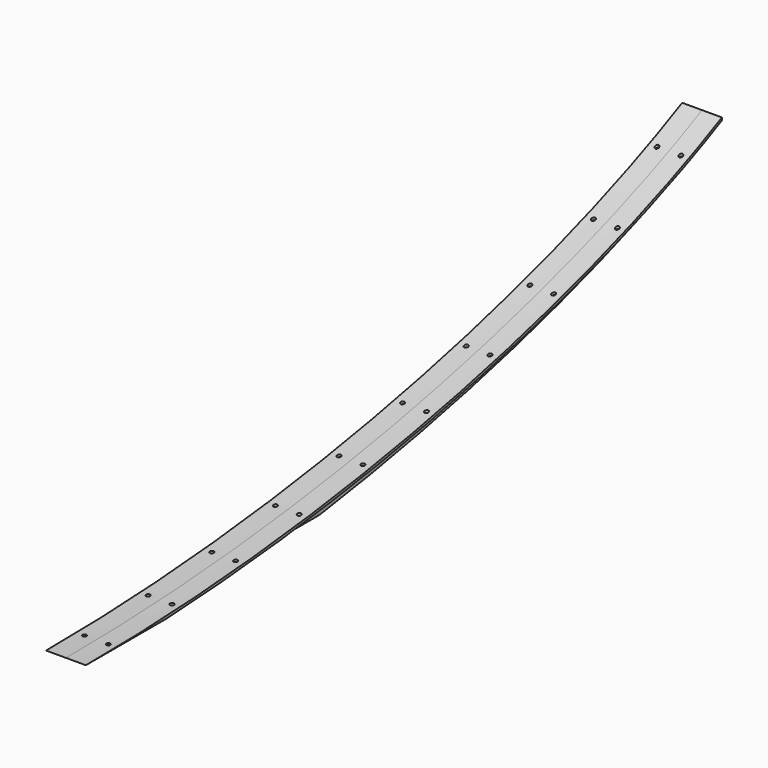
from build123d import *

# Parameters (mm, degrees)
F1_DEPTH = 25
F2_DEPTH = 4.5
F3_DEPTH = 1.5
F4_R     = 2.5
F5_DEPTH = 150
F6_R     = 4.1800646045
F7_DEPTH = 12.5


# Not quite as in the source:
# - the dataset's text gives a spline's control points without its knots; the knots are read off the source's solid


with BuildPart() as f1:
    # F0 (on Right) → F1 (new body, symmetric)
    with BuildSketch(Plane.YZ):
        with BuildLine():
            add(Edge.make_bspline(
                [(-542.9529296271, -39.9508323044), (-188.0693441655, -39.9508323044), (204.5968802247, 34.2876766354), (457.0470703729, 160.0491676956)],
                knots=[0, 0, 0, 0, 1019.8039027186, 1019.8039027186, 1019.8039027186, 1019.8039027186], degree=3))
            Line((-542.9529296271, -39.9508323044), (-417.3127151335, -39.9508323044))
            add(Edge.make_bspline(
                [(-417.3127151335, -39.9508323044), (-369.1001563129, -37.6799090107), (-229.605831227, -27.4883990926), (-0.7659143619, 6.0089411279), (250.4802761754, 69.14721948), (394.0857076642, 125.4398419701), (457.047070373, 156.6986558412)],
                knots=[0.116693999, 0.116693999, 0.116693999, 0.116693999, 0.25, 0.5, 0.75, 0.9982402372, 0.9982402372, 0.9982402372, 0.9982402372], degree=3))
            Line((457.0470703729, 156.6986558412), (457.0470703729, 160.0491676956))
        make_face()
    extrude(amount=F1_DEPTH, both=True)

    # F0 (on Right) → F2 (join, symmetric)
    with BuildSketch(Plane.YZ):
        with BuildLine():
            add(Edge.make_bspline(
                [(-417.3127151335, -39.9508323044), (-369.1001563129, -37.6799090107), (-229.605831227, -27.4883990926), (-0.7659143619, 6.0089411279), (250.4802761754, 69.14721948), (394.0857076642, 125.4398419701), (457.047070373, 156.6986558412)],
                knots=[0.116693999, 0.116693999, 0.116693999, 0.116693999, 0.25, 0.5, 0.75, 0.9982402372, 0.9982402372, 0.9982402372, 0.9982402372], degree=3))
            Line((-417.3127151335, -39.9508323044), (-149.937543661, -39.9508323044))
            add(Edge.make_bspline(
                [(-149.937543661, -39.9508323044), (-98.996798705, -32.7943859429), (-3.7016307054, -16.778446645), (131.246444394, 13.3933570474), (254.1058325956, 48.1234806847), (363.3774188375, 86.6936370443), (428.3490574687, 114.995507991), (457.0470703729, 128.861665731)],
                knots=[0.3594995159, 0.3594995159, 0.3594995159, 0.3594995159, 0.5, 0.625, 0.75, 0.875, 0.9840561675, 0.9840561675, 0.9840561675, 0.9840561675], degree=3))
            Line((457.0470703729, 128.861665731), (457.0470703729, 156.6986558412))
        make_face()
    extrude(amount=F2_DEPTH, both=True)

    # F0 (on Right) → F3 (cut, symmetric)
    with BuildSketch(Plane.YZ):
        with BuildLine():
            add(Edge.make_bspline(
                [(-417.3127151335, -39.9508323044), (-369.1001563129, -37.6799090107), (-229.605831227, -27.4883990926), (-0.7659143619, 6.0089411279), (250.4802761754, 69.14721948), (394.0857076642, 125.4398419701), (457.047070373, 156.6986558412)],
                knots=[0.116693999, 0.116693999, 0.116693999, 0.116693999, 0.25, 0.5, 0.75, 0.9982402372, 0.9982402372, 0.9982402372, 0.9982402372], degree=3))
            Line((-417.3127151335, -39.9508323044), (-149.937543661, -39.9508323044))
            add(Edge.make_bspline(
                [(-149.937543661, -39.9508323044), (-98.996798705, -32.7943859429), (-3.7016307054, -16.778446645), (131.246444394, 13.3933570474), (254.1058325956, 48.1234806847), (363.3774188375, 86.6936370443), (428.3490574687, 114.995507991), (457.0470703729, 128.861665731)],
                knots=[0.3594995159, 0.3594995159, 0.3594995159, 0.3594995159, 0.5, 0.625, 0.75, 0.875, 0.9840561675, 0.9840561675, 0.9840561675, 0.9840561675], degree=3))
            Line((457.0470703729, 128.861665731), (457.0470703729, 156.6986558412))
        make_face()
    extrude(amount=F3_DEPTH, both=True, mode=Mode.SUBTRACT)

    # F4 (on Top) → F5 (cut, symmetric)
    with BuildSketch(Plane.XY):
        with Locations((15, -494.9529296271)):
            Circle(F4_R)
        with Locations((15, -394.9529296271)):
            Circle(F4_R)
        with Locations((15, -294.9529296271)):
            Circle(F4_R)
        with Locations((15, -194.9529296271)):
            Circle(F4_R)
        with Locations((15, -94.9529296271)):
            Circle(F4_R)
        with Locations((15, 5.0470703729)):
            Circle(F4_R)
        with Locations((15, 105.0470703729)):
            Circle(F4_R)
        with Locations((15, 205.0470703729)):
            Circle(F4_R)
        with Locations((15, 305.0470703729)):
            Circle(F4_R)
        with Locations((15, 405.0470703729)):
            Circle(F4_R)
        with Locations((-15, -494.9529296271)):
            Circle(F4_R)
        with Locations((-15, -394.9529296271)):
            Circle(F4_R)
        with Locations((-15, -294.9529296271)):
            Circle(F4_R)
        with Locations((-15, -194.9529296271)):
            Circle(F4_R)
        with Locations((-15, -94.9529296271)):
            Circle(F4_R)
        with Locations((-15, 5.0470703729)):
            Circle(F4_R)
        with Locations((-15, 105.0470703729)):
            Circle(F4_R)
        with Locations((-15, 205.0470703729)):
            Circle(F4_R)
        with Locations((-15, 305.0470703729)):
            Circle(F4_R)
        with Locations((-15, 405.0470703729)):
            Circle(F4_R)
    extrude(amount=F5_DEPTH, both=True, mode=Mode.SUBTRACT)

    # F6 (on Right) → F7 (cut, symmetric)
    with BuildSketch(Plane.YZ):
        with Locations((442.0470703729, 131.861665731)):
            Circle(F6_R)
        with Locations((358.44841201, 95.9379511725)):
            Circle(F6_R)
        with Locations((273.163023997, 64.2259417875)):
            Circle(F6_R)
        with Locations((186.4029392463, 36.8044786279)):
            Circle(F6_R)
        with Locations((98.3838569987, 13.7417357717)):
            Circle(F6_R)
        with Locations((9.3246065611, -4.9049491686)):
            Circle(F6_R)
        with Locations((-80.5533967375, -19.0892175961)):
            Circle(F6_R)
        with Locations((-171.0267020195, -28.7758051847)):
            Circle(F6_R)
    extrude(amount=F7_DEPTH, both=True, mode=Mode.SUBTRACT)


solid = f1.part
